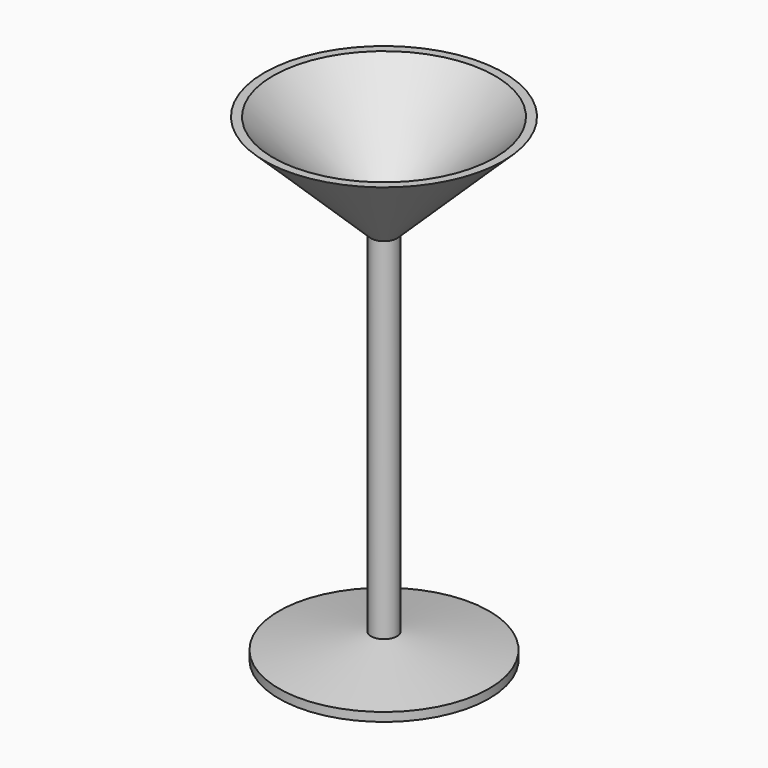
from build123d import *

# Parameters (mm, degrees)
F2_T = 2.5


# Not quite as in the source:
# - a shell that OpenCascade refuses in one call is made with other operations: the cavity is built on its own and cut out


with BuildPart() as f1:
    # F0 (on Front) → F1 (revolve)
    with BuildSketch(Plane.XZ):
        Polygon((0, 98.8223368999), (0, -101.1776631001), (43.9656563103, -101.1776631001), (43.9656563103, -97.5007638335), (5.4530212656, -90.7485485077), (5.4530212656, 55.7995252311), (50, 98.8223368999), align=None)
    revolve(axis=Axis((0, 0, -1.1776631001), (0, 0, 1)))

    # F2: shell of thickness 2.5, made by hand


with BuildPart() as f2_core1:
    # F2_t2: copy of F1
    add(f1.part)

    # the walls: a layer under each face that stays
    f2_faces = [f2_core1.faces().sort_by_distance(p)[0] for p in [
        (-27.7265106328, 0, 77.3109310655),
        (0, 0, -101.1776631001),
        (-43.9656563103, 0, -99.3392134668),
        (-24.7093387879, 0, -94.1246561706),
        (-5.4530212656, 0, -17.4745116383),
    ]]
    thicken(f2_faces, amount=-F2_T, mode=Mode.SUBTRACT)

    # F2_s3 → F2_t4 (revolve, cut)
    with BuildSketch(Plane.XZ):
        Polygon((5.4953886218, 55.7815426024), (3.7162856398, 57.5977881058), (2.9530212656, 56.8606386882), (2.9530212656, 55.7995252311), align=None)
    revolve(axis=Axis((0, 0, 55.7995252311), (0, 0, 1)), mode=Mode.SUBTRACT)

    # F2_s5 → F2_t6 (revolve, cut)
    with BuildSketch(Plane.XZ):
        Polygon((5.4823385311, -90.7239241048), (5.0212947153, -93.2109887985), (2.9530212656, -92.8483694226), (2.9530212656, -90.7485485077), align=None)
    revolve(axis=Axis((0, 0, -90.7485485077), (0, 0, 1)), mode=Mode.SUBTRACT)


with BuildPart() as f1_1:
    add(f1.part)

    # what is left inside the walls is the cavity
    f2_cavity = [f2_core1.part.solids().sort_by_distance(p)[0] for p in [
        (-17.927255, 0, 71.357287),
    ]]
    add(f2_cavity, mode=Mode.SUBTRACT)


solid = f1_1.part
